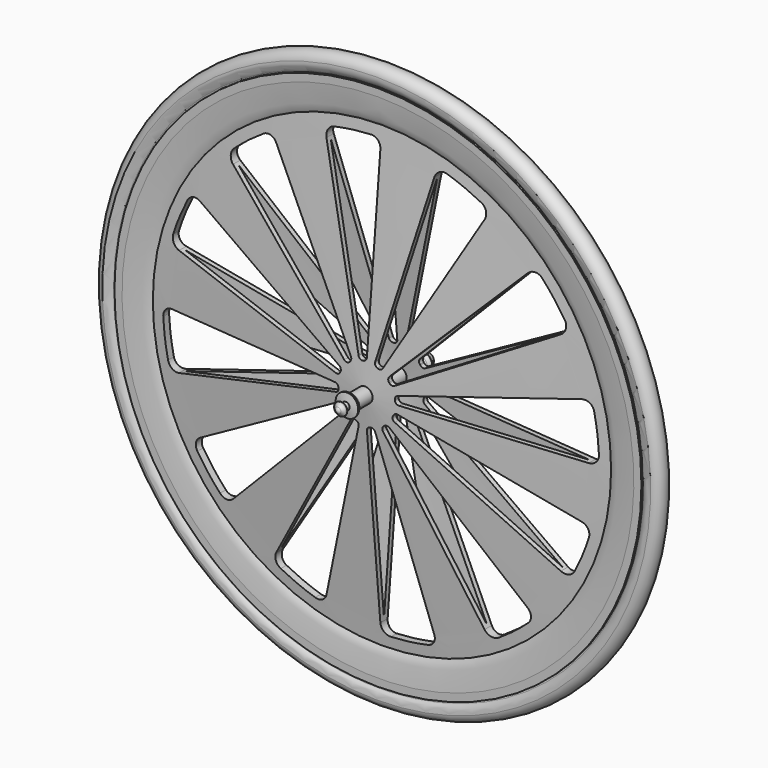
from build123d import *

# Parameters (mm, degrees)
F5_DEPTH = 37.592


with BuildPart() as f1:
    # F0 (on Right) → F1 (revolve)
    with BuildSketch(Plane.YZ):
        with BuildLine():
            Line((71.501, 7.5438), (71.501, 5.0038))
            Line((71.501, 5.0038), (63.881, 5.0038))
            Line((63.881, 5.0038), (62.089517876, 15.1638))
            ThreePointArc((62.089517876, 15.1638), (59.3166092052, 14.4173787383), (57.2930966272, 12.3798400164))
            ThreePointArc((57.2930966272, 12.3798400164), (55.6242271464, 10.6994026294), (53.3373015773, 10.0838))
            Line((53.3373015773, 10.0838), (0, 10.0838))
            Line((0, 10.0838), (-53.3373015773, 10.0838))
            ThreePointArc((-53.3373015773, 10.0838), (-55.6242271464, 10.6994026294), (-57.2930966272, 12.3798400164))
            ThreePointArc((-57.2930966272, 12.3798400164), (-59.3166092052, 14.4173787383), (-62.089517876, 15.1638))
            Line((-62.089517876, 15.1638), (-63.881, 5.0038))
            Line((-63.881, 5.0038), (-71.501, 5.0038))
            Line((-71.501, 5.0038), (-71.501, 7.5438))
            ThreePointArc((-71.501, 7.5438), (-72.2497323653, 8.5240163085), (-73.3923858493, 8.059508847))
            ThreePointArc((-73.3923858493, 8.059508847), (-75.0412667877, 5.8185715621), (-77.1098260384, 3.9580149543))
            ThreePointArc((-77.1098260384, 3.9580149543), (-78.5893682281, 2.2198368793), (-79.121, 0))
            Line((-79.121, 0), (0, 0))
            Line((0, 0), (79.121, 0))
            ThreePointArc((79.121, 0), (78.5893682281, 2.2198368793), (77.1098260384, 3.9580149543))
            ThreePointArc((77.1098260384, 3.9580149543), (75.0412667877, 5.8185715621), (73.3923858493, 8.059508847))
            ThreePointArc((73.3923858493, 8.059508847), (72.2497323653, 8.5240163085), (71.501, 7.5438))
        make_face()
    revolve(axis=Axis((0, -39.5605, 0), (0, -1, 0)))


with BuildPart() as f3:
    # F2 (on Right) → F3 (revolve)
    with BuildSketch(Plane.YZ):
        with BuildLine():
            Line((-6.35, 346.6338), (6.35, 346.6338))
            ThreePointArc((6.35, 346.6338), (6.8514798128, 351.0985723649), (9.0096217384, 355.0391430979))
            ThreePointArc((9.0096217384, 355.0391430979), (12.070667246, 360.7600413514), (12.6059821495, 367.2262701117))
            ThreePointArc((12.6059821495, 367.2262701117), (0, 378.3838), (-12.6059821495, 367.2262701117))
            ThreePointArc((-12.6059821495, 367.2262701117), (-12.070667246, 360.7600413514), (-9.0096217384, 355.0391430979))
            ThreePointArc((-9.0096217384, 355.0391430979), (-6.8514798128, 351.0985723649), (-6.35, 346.6338))
        make_face()
    revolve(axis=Axis((0, 53.3373015773, 0), (0, -1, 0)))


with BuildPart() as f3b:
    # F2 (on Right) → F3, piece 2 (revolve)
    with BuildSketch(Plane.YZ):
        with BuildLine():
            Line((0, 342.7984), (10.16, 342.7984))
            Line((10.16, 342.7984), (10.16, 352.9584))
            Line((10.16, 352.9584), (7.6516344269, 352.9584))
            ThreePointArc((7.6516344269, 352.9584), (6.5621274424, 349.8741862214), (6.3776268799, 346.6084))
            Line((6.3776268799, 346.6084), (-6.3776268799, 346.6084))
            ThreePointArc((-6.3776268799, 346.6084), (-6.5621274424, 349.8741862214), (-7.6516344269, 352.9584))
            Line((-7.6516344269, 352.9584), (-10.16, 352.9584))
            Line((-10.16, 352.9584), (-10.16, 342.7984))
            Line((-10.16, 342.7984), (0, 342.7984))
        make_face()
        with BuildLine():
            add(Edge.make_bspline(
                [(-10.16, 342.7984), (-10.16, 315.9665152576), (-3.4231911955, 306.9260948236)],
                knots=[1.5707963268, 1.5707963268, 1.5707963268, 2.797940158, 2.797940158, 2.797940158], degree=2, weights=[1, 0.8175965592, 1]))
            Line((-3.4231911956, 306.9260948236), (0, 342.7984))
            Line((0, 342.7984), (-10.16, 342.7984))
        make_face()
        with BuildLine():
            Line((0, 342.7984), (3.4231911956, 306.9260948236))
            add(Edge.make_bspline(
                [(3.4231911955, 306.9260948236), (10.16, 315.9665152576), (10.16, 342.7984)],
                knots=[3.4852451492, 3.4852451492, 3.4852451492, 4.7123889804, 4.7123889804, 4.7123889804], degree=2, weights=[1, 0.8175965592, 1]))
            Line((10.16, 342.7984), (0, 342.7984))
        make_face()
        with BuildLine():
            Line((25.3711524303, 10.0838), (26.6686507886, 10.0838))
            Line((26.6686507886, 10.0838), (31.75, 10.0838))
            Line((31.75, 10.0838), (3.4231911956, 306.9260948236))
            add(Edge.make_bspline(
                [(-3.4231911955, 306.9260948236), (0, 302.3323637957), (3.4231911955, 306.9260948236)],
                knots=[2.797940158, 2.797940158, 2.797940158, 3.4852451492, 3.4852451492, 3.4852451492], degree=2, weights=[1, 0.9415303196, 1]))
            Line((-3.4231911956, 306.9260948236), (-31.75, 10.0838))
            Line((-31.75, 10.0838), (-25.3711524303, 10.0838))
            Line((-25.3711524303, 10.0838), (0, 275.9531805478))
            Line((0, 275.9531805478), (25.3711524303, 10.0838))
        make_face()
        with BuildLine():
            add(Edge.make_bspline(
                [(-3.4231911955, 306.9260948236), (0, 302.3323637957), (3.4231911955, 306.9260948236)],
                knots=[2.797940158, 2.797940158, 2.797940158, 3.4852451492, 3.4852451492, 3.4852451492], degree=2, weights=[1, 0.9415303196, 1]))
            Line((3.4231911956, 306.9260948236), (0, 342.7984))
            Line((0, 342.7984), (-3.4231911956, 306.9260948236))
        make_face()
    revolve(axis=Axis((0, 53.3373015773, 0), (0, -1, 0)))

    # F4 (on Front) → F5 (cut, symmetric)
    with BuildSketch(Plane.XZ):
        with BuildLine():
            ThreePointArc((-4.4823529412, 37.8354134656), (-1.2824713919, 39.5059425471), (0, 42.880135261))
            Line((0, 42.880135261), (0, 279.1112143931))
            ThreePointArc((0, 279.1112143931), (-3.9262141477, 288.2932992227), (-13.2772727273, 291.7980877746))
            ThreePointArc((-13.2772727273, 291.7980877746), (-38.1267007475, 289.6010440073), (-62.6980418106, 285.2917200921))
            ThreePointArc((-62.6980418106, 285.2917200921), (-70.8233647695, 279.4861222619), (-72.2392979866, 269.6007303892))
            Line((-72.2392979866, 269.6007303892), (-11.0981956621, 41.4190300833))
            ThreePointArc((-11.0981956621, 41.4190300833), (-8.986118087, 38.4917382191), (-5.4629051158, 37.7063213228))
            ThreePointArc((-5.4629051158, 37.7063213228), (-4.9730479236, 37.7740492183), (-4.4823529412, 37.8354134656))
        make_face()
        with BuildLine():
            Line((-197.3614324026, 197.3614324026), (-30.3208344212, 30.3208344212))
            ThreePointArc((-30.3208344212, 30.3208344212), (-27.0280756543, 28.8417640901), (-23.5841752701, 29.9231795909))
            ThreePointArc((-23.5841752701, 29.9231795909), (-23.1938104452, 30.2267622651), (-22.7995382486, 30.5252527533))
            ThreePointArc((-22.7995382486, 30.5252527533), (-20.8636240785, 33.5719141503), (-21.4400676305, 37.1352864537))
            Line((-21.4400676305, 37.1352864537), (-139.5556071966, 241.7174021456))
            ThreePointArc((-139.5556071966, 241.7174021456), (-147.546850804, 247.7062137939), (-157.3974993621, 246.0659204249))
            ThreePointArc((-157.3974993621, 246.0659204249), (-177.8192134134, 231.7385106991), (-196.9439570216, 215.7208561838))
            ThreePointArc((-196.9439570216, 215.7208561838), (-201.0778942028, 206.6303994993), (-197.3614324026, 197.3614324026))
        make_face()
        with BuildLine():
            Line((-269.6007303892, 72.2392979866), (-41.4190300833, 11.0981956621))
            ThreePointArc((-41.4190300833, 11.0981956621), (-37.8278821771, 11.4636625648), (-35.3860847067, 14.1221460526))
            ThreePointArc((-35.3860847067, 14.1221460526), (-35.1998101887, 14.5802387731), (-35.0076056945, 15.035875217))
            ThreePointArc((-35.0076056945, 15.035875217), (-34.8543855422, 18.6423184685), (-37.1352864537, 21.4400676305))
            Line((-37.1352864537, 21.4400676305), (-241.7174021456, 139.5556071966))
            ThreePointArc((-241.7174021456, 139.5556071966), (-251.6324279416, 140.7464484187), (-259.3431931522, 134.4005884125))
            ThreePointArc((-259.3431931522, 134.4005884125), (-269.8652114465, 111.7818305938), (-278.4188979944, 88.3477630705))
            ThreePointArc((-278.4188979944, 88.3477630705), (-277.4537642687, 78.4082280591), (-269.6007303892, 72.2392979866))
        make_face()
        with BuildLine():
            Line((-269.6007303892, -72.2392979866), (-41.4190300833, -11.0981956621))
            ThreePointArc((-41.4190300833, -11.0981956621), (-38.4917382191, -8.986118087), (-37.7063213228, -5.4629051158))
            ThreePointArc((-37.7063213228, -5.4629051158), (-37.7740492183, -4.9730479236), (-37.8354134656, -4.4823529412))
            ThreePointArc((-37.8354134656, -4.4823529412), (-39.5059425471, -1.2824713919), (-42.880135261, 0))
            Line((-42.880135261, 0), (-279.1112143931, 0))
            ThreePointArc((-279.1112143931, 0), (-288.2932992227, -3.9262141477), (-291.7980877746, -13.2772727273))
            ThreePointArc((-291.7980877746, -13.2772727273), (-289.6010440073, -38.1267007475), (-285.2917200921, -62.6980418106))
            ThreePointArc((-285.2917200921, -62.6980418106), (-279.4861222619, -70.8233647695), (-269.6007303892, -72.2392979866))
        make_face()
        with BuildLine():
            Line((-197.3614324026, -197.3614324026), (-30.3208344212, -30.3208344212))
            ThreePointArc((-30.3208344212, -30.3208344212), (-28.8417640901, -27.0280756543), (-29.9231795909, -23.5841752701))
            ThreePointArc((-29.9231795909, -23.5841752701), (-30.2267622651, -23.1938104452), (-30.5252527533, -22.7995382486))
            ThreePointArc((-30.5252527533, -22.7995382486), (-33.5719141503, -20.8636240785), (-37.1352864537, -21.4400676305))
            Line((-37.1352864537, -21.4400676305), (-241.7174021456, -139.5556071966))
            ThreePointArc((-241.7174021456, -139.5556071966), (-247.7062137939, -147.546850804), (-246.0659204249, -157.3974993621))
            ThreePointArc((-246.0659204249, -157.3974993621), (-231.7385106991, -177.8192134134), (-215.7208561838, -196.9439570216))
            ThreePointArc((-215.7208561838, -196.9439570216), (-206.6303994993, -201.0778942028), (-197.3614324026, -197.3614324026))
        make_face()
        with BuildLine():
            Line((-72.2392979866, -269.6007303892), (-11.0981956621, -41.4190300833))
            ThreePointArc((-11.0981956621, -41.4190300833), (-11.4636625648, -37.8278821771), (-14.1221460526, -35.3860847067))
            ThreePointArc((-14.1221460526, -35.3860847067), (-14.5802387731, -35.1998101887), (-15.035875217, -35.0076056945))
            ThreePointArc((-15.035875217, -35.0076056945), (-18.6423184685, -34.8543855422), (-21.4400676305, -37.1352864537))
            Line((-21.4400676305, -37.1352864537), (-139.5556071966, -241.7174021456))
            ThreePointArc((-139.5556071966, -241.7174021456), (-140.7464484187, -251.6324279416), (-134.4005884125, -259.3431931522))
            ThreePointArc((-134.4005884125, -259.3431931522), (-111.7818305938, -269.8652114465), (-88.3477630705, -278.4188979944))
            ThreePointArc((-88.3477630705, -278.4188979944), (-78.4082280591, -277.4537642687), (-72.2392979866, -269.6007303892))
        make_face()
        with BuildLine():
            Line((72.2392979866, -269.6007303892), (11.0981956621, -41.4190300833))
            ThreePointArc((11.0981956621, -41.4190300833), (8.986118087, -38.4917382191), (5.4629051158, -37.7063213228))
            ThreePointArc((5.4629051158, -37.7063213228), (4.9730479236, -37.7740492183), (4.4823529412, -37.8354134656))
            ThreePointArc((4.4823529412, -37.8354134656), (1.2824713919, -39.5059425471), (0, -42.880135261))
            Line((0, -42.880135261), (0, -279.1112143931))
            ThreePointArc((0, -279.1112143931), (3.9262141477, -288.2932992227), (13.2772727273, -291.7980877746))
            ThreePointArc((13.2772727273, -291.7980877746), (38.1267007475, -289.6010440073), (62.6980418106, -285.2917200921))
            ThreePointArc((62.6980418106, -285.2917200921), (70.8233647695, -279.4861222619), (72.2392979866, -269.6007303892))
        make_face()
        with BuildLine():
            Line((197.3614324026, -197.3614324026), (30.3208344212, -30.3208344212))
            ThreePointArc((30.3208344212, -30.3208344212), (27.0280756543, -28.8417640901), (23.5841752701, -29.9231795909))
            ThreePointArc((23.5841752701, -29.9231795909), (23.1938104452, -30.2267622651), (22.7995382486, -30.5252527533))
            ThreePointArc((22.7995382486, -30.5252527533), (20.8636240785, -33.5719141503), (21.4400676305, -37.1352864537))
            Line((21.4400676305, -37.1352864537), (139.5556071966, -241.7174021456))
            ThreePointArc((139.5556071966, -241.7174021456), (147.546850804, -247.7062137939), (157.3974993621, -246.0659204249))
            ThreePointArc((157.3974993621, -246.0659204249), (177.8192134134, -231.7385106991), (196.9439570216, -215.7208561838))
            ThreePointArc((196.9439570216, -215.7208561838), (201.0778942028, -206.6303994993), (197.3614324026, -197.3614324026))
        make_face()
        with BuildLine():
            Line((269.6007303892, -72.2392979866), (41.4190300833, -11.0981956621))
            ThreePointArc((41.4190300833, -11.0981956621), (37.8278821771, -11.4636625648), (35.3860847067, -14.1221460526))
            ThreePointArc((35.3860847067, -14.1221460526), (35.1998101887, -14.5802387731), (35.0076056945, -15.035875217))
            ThreePointArc((35.0076056945, -15.035875217), (34.8543855422, -18.6423184685), (37.1352864537, -21.4400676305))
            Line((37.1352864537, -21.4400676305), (241.7174021456, -139.5556071966))
            ThreePointArc((241.7174021456, -139.5556071966), (251.6324279416, -140.7464484187), (259.3431931522, -134.4005884125))
            ThreePointArc((259.3431931522, -134.4005884125), (269.8652114465, -111.7818305938), (278.4188979944, -88.3477630705))
            ThreePointArc((278.4188979944, -88.3477630705), (277.4537642687, -78.4082280591), (269.6007303892, -72.2392979866))
        make_face()
        with BuildLine():
            Line((269.6007303892, 72.2392979866), (41.4190300833, 11.0981956621))
            ThreePointArc((41.4190300833, 11.0981956621), (38.4917382191, 8.986118087), (37.7063213228, 5.4629051158))
            ThreePointArc((37.7063213228, 5.4629051158), (37.7740492183, 4.9730479236), (37.8354134656, 4.4823529412))
            ThreePointArc((37.8354134656, 4.4823529412), (39.5059425471, 1.2824713919), (42.880135261, 0))
            Line((42.880135261, 0), (279.1112143931, 0))
            ThreePointArc((279.1112143931, 0), (288.2932992227, 3.9262141477), (291.7980877746, 13.2772727273))
            ThreePointArc((291.7980877746, 13.2772727273), (289.6010440073, 38.1267007475), (285.2917200921, 62.6980418106))
            ThreePointArc((285.2917200921, 62.6980418106), (279.4861222619, 70.8233647695), (269.6007303892, 72.2392979866))
        make_face()
        with BuildLine():
            Line((197.3614324026, 197.3614324026), (30.3208344212, 30.3208344212))
            ThreePointArc((30.3208344212, 30.3208344212), (28.8417640901, 27.0280756543), (29.9231795909, 23.5841752701))
            ThreePointArc((29.9231795909, 23.5841752701), (30.2267622651, 23.1938104452), (30.5252527533, 22.7995382486))
            ThreePointArc((30.5252527533, 22.7995382486), (33.5719141503, 20.8636240785), (37.1352864537, 21.4400676305))
            Line((37.1352864537, 21.4400676305), (241.7174021456, 139.5556071966))
            ThreePointArc((241.7174021456, 139.5556071966), (247.7062137939, 147.546850804), (246.0659204249, 157.3974993621))
            ThreePointArc((246.0659204249, 157.3974993621), (231.7385106991, 177.8192134134), (215.7208561838, 196.9439570216))
            ThreePointArc((215.7208561838, 196.9439570216), (206.6303994993, 201.0778942028), (197.3614324026, 197.3614324026))
        make_face()
        with BuildLine():
            Line((72.2392979866, 269.6007303892), (11.0981956621, 41.4190300833))
            ThreePointArc((11.0981956621, 41.4190300833), (11.4636625648, 37.8278821771), (14.1221460526, 35.3860847067))
            ThreePointArc((14.1221460526, 35.3860847067), (14.5802387731, 35.1998101887), (15.035875217, 35.0076056945))
            ThreePointArc((15.035875217, 35.0076056945), (18.6423184685, 34.8543855422), (21.4400676305, 37.1352864537))
            Line((21.4400676305, 37.1352864537), (139.5556071966, 241.7174021456))
            ThreePointArc((139.5556071966, 241.7174021456), (140.7464484187, 251.6324279416), (134.4005884125, 259.3431931522))
            ThreePointArc((134.4005884125, 259.3431931522), (111.7818305938, 269.8652114465), (88.3477630705, 278.4188979944))
            ThreePointArc((88.3477630705, 278.4188979944), (78.4082280591, 277.4537642687), (72.2392979866, 269.6007303892))
        make_face()
    extrude(amount=F5_DEPTH, both=True, mode=Mode.SUBTRACT)


solid = Compound([f1.part, f3.part, f3b.part])
